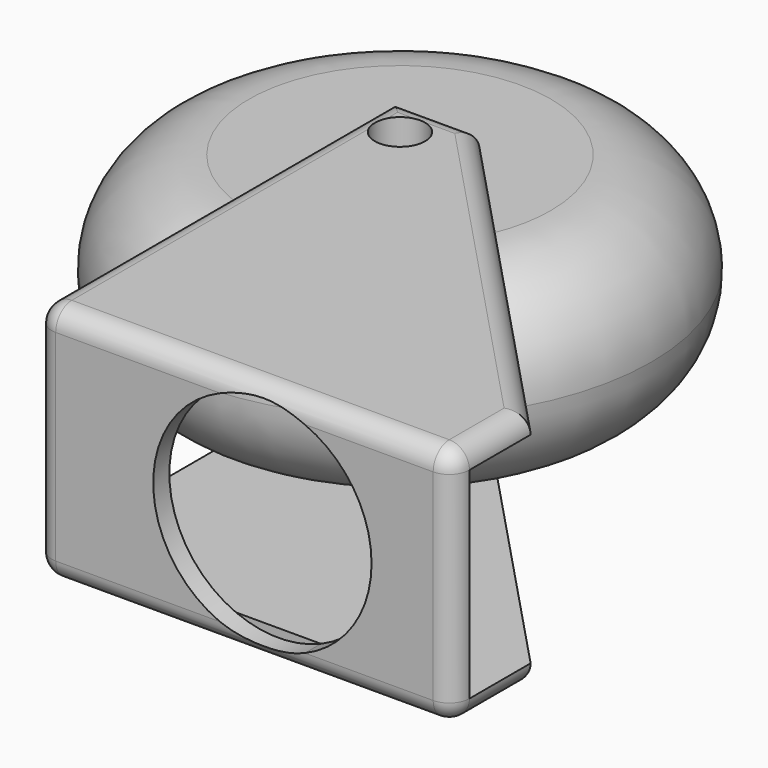
from build123d import *

# Parameters (mm, degrees)
F0_R          = 25
F1_DEPTH      = 20
F2_R          = 9.99999
F3_R          = 2.5
F4_DEPTH      = 25.4
F5_R          = 2.5
F6_DEPTH      = 2
F7_W          = 41.5132804774
F7_H          = 2
F8_DEPTH      = 20
F9_R          = 2.5
F9_W          = 41.5132804774
F9_H          = 2
F10_DEPTH     = 2
F11_T1_DEPTH  = 20
F11_T3_DEPTH  = 47.4638193212
F11_T5_DEPTH  = 37.5132804774
F11_T7_DEPTH  = 12.6040666103
F11_T9_DEPTH  = 57.9730332998
F11_T11_DEPTH = 18.5555869155
F11_T13_DEPTH = 57.9730332998
F11_S17_W     = 2
F11_S17_H     = 2
F11_T18_DEPTH = 2
F11_S23_W     = 2
F11_S23_H     = 2
F11_T24_DEPTH = 2
F11_S29_W     = 2
F11_S29_H     = 2
F11_T30_DEPTH = 2
F11_S35_W     = 2
F11_S35_H     = 2
F11_T36_DEPTH = 2
F13_DEPTH     = 2


# Not quite as in the source:
# - a fillet or chamfer that OpenCascade refuses, or shapes differently, is made with other operations: its cross-section is extruded or revolved along the edge and cut away or added
# - a fillet or chamfer is up to 0.001 mm smaller than in the source, because OpenCascade refuses the exact size


with BuildPart() as f1:
    # F0 (on Top) → F1 (new body)
    with BuildSketch(Plane.XY):
        Circle(F0_R)
    extrude(amount=F1_DEPTH)

    # F2 (radius 10 in the source; OpenCascade refuses exactly that, so slightly less here)
    f2_edges = [f1.edges().sort_by_distance(p)[0] for p in [
        (-25, 0, 20),
        (-25, 0, 0),
    ]]
    fillet(f2_edges, radius=F2_R)

    # F3 (on face) → F4 (cut)
    with BuildSketch(Plane.XY.offset(20)):
        Circle(F3_R)
    extrude(amount=-F4_DEPTH, mode=Mode.SUBTRACT)

    # F5 (on face) → F6 (join)
    with BuildSketch(Plane(origin=(0, 0, 0), x_dir=(1, 0, 0), z_dir=(0, 0, -1))):
        with BuildLine():
            Line((37.3017899692, 30.3959333897), (37.3017899692, 40))
            Line((37.3017899692, 40), (-4.2114905082, 40))
            Line((-4.2114905082, 40), (-4.2114905082, 14.3966540453))
            ThreePointArc((-4.2114905082, 14.3966540453), (6.5284436355, 13.5048037268), (13.8984988304, 5.641988148))
            Line((13.8984988304, 5.641988148), (37.3017899692, 30.3959333897))
        make_face()
        with BuildLine():
            Line((4.3440964073, -4.4638193212), (13.8984988304, 5.641988148))
            ThreePointArc((13.8984988304, 5.641988148), (6.5284436355, 13.5048037268), (-4.2114905082, 14.3966540453))
            Line((-4.2114905082, 14.3966540453), (-4.2114905082, -4.4638193212))
            Line((-4.2114905082, -4.4638193212), (4.3440964073, -4.4638193212))
        make_face()
        Circle(F5_R, mode=Mode.SUBTRACT)
    extrude(amount=F6_DEPTH)

    # F7 (on face) → F8 (join)
    with BuildSketch(Plane.XY):
        with Locations((16.5451497305, -39)):
            Rectangle(F7_W, F7_H)
    extrude(amount=F8_DEPTH)

    # F9 (on face) → F10 (join)
    with BuildSketch(Plane.XY.offset(20)):
        Polygon((37.3017899692, -38), (37.3017899692, -30.3959333897), (4.3440964073, 4.4638193212), (-4.2114905082, 4.4638193212), (-4.2114905082, -38), align=None)
        Circle(F9_R, mode=Mode.SUBTRACT)
        with Locations((16.5451497305, -39)):
            Rectangle(F9_W, F9_H)
    extrude(amount=F10_DEPTH)

    # F11: fillet of radius 2 on 12 edges, made by hand

    # F11_s2 → F11_t1 (cut)
    with BuildSketch(Plane.XY):
        with BuildLine():
            ThreePointArc((-2.2114905082, -40), (-3.6257040705, -39.4142135624), (-4.2114905082, -38))
            Line((-4.2114905082, -38), (-4.2114905082, -40))
            Line((-4.2114905082, -40), (-2.2114905082, -40))
        make_face()
        with BuildLine():
            ThreePointArc((35.3017899692, -40), (36.7160035316, -39.4142135624), (37.3017899692, -38))
            Line((37.3017899692, -38), (37.3017899692, -40))
            Line((37.3017899692, -40), (35.3017899692, -40))
        make_face()
    extrude(amount=F11_T1_DEPTH, mode=Mode.SUBTRACT)

    # F11_s4 → F11_t3 (cut)
    with BuildSketch(Plane.XZ.offset(-9.4638193212)):
        with BuildLine():
            ThreePointArc((-2.2114905082, 22), (-3.6257040705, 21.4142135624), (-4.2114905082, 20))
            Line((-4.2114905082, 20), (-4.2114905082, 22))
            Line((-4.2114905082, 22), (-2.2114905082, 22))
        make_face()
        with BuildLine():
            ThreePointArc((-2.2114905082, -2), (-3.6257040705, -1.4142135624), (-4.2114905082, 0))
            Line((-4.2114905082, 0), (-4.2114905082, -2))
            Line((-4.2114905082, -2), (-2.2114905082, -2))
        make_face()
    extrude(amount=F11_T3_DEPTH, mode=Mode.SUBTRACT)

    # F11_s6 → F11_t5 (cut)
    with BuildSketch(Plane.YZ.offset(-2.2114905082)):
        with BuildLine():
            ThreePointArc((-38, 22), (-39.4142135624, 21.4142135624), (-40, 20))
            Line((-40, 20), (-40, 22))
            Line((-40, 22), (-38, 22))
        make_face()
        with BuildLine():
            ThreePointArc((-38, -2), (-39.4142135624, -1.4142135624), (-40, 0))
            Line((-40, 0), (-40, -2))
            Line((-40, -2), (-38, -2))
        make_face()
    extrude(amount=F11_T5_DEPTH, mode=Mode.SUBTRACT)

    # F11_s8 → F11_t7 (cut)
    with BuildSketch(Plane.XZ.offset(25.3959333897)):
        with BuildLine():
            ThreePointArc((35.3017899692, 22), (36.7160035316, 21.4142135624), (37.3017899692, 20))
            Line((37.3017899692, 20), (37.3017899692, 22))
            Line((37.3017899692, 22), (35.3017899692, 22))
        make_face()
        with BuildLine():
            ThreePointArc((35.3017899692, -2), (36.7160035316, -1.4142135624), (37.3017899692, 0))
            Line((37.3017899692, 0), (37.3017899692, -2))
            Line((37.3017899692, -2), (35.3017899692, -2))
        make_face()
    extrude(amount=F11_T7_DEPTH, mode=Mode.SUBTRACT)

    # F11_s10 → F11_t9 (cut)
    with BuildSketch(Plane(origin=(36.2146215396, -38.3046449843, 0), x_dir=(0, 0, 1), z_dir=(-0.6870045793, 0.7266530864, 0))):
        with BuildLine():
            ThreePointArc((20, 6.223315377), (21.4142135624, 5.6375289394), (22, 4.223315377))
            Line((22, 4.223315377), (22, 6.223315377))
            Line((22, 6.223315377), (20, 6.223315377))
        make_face()
    extrude(amount=F11_T9_DEPTH, mode=Mode.SUBTRACT)

    # F11_s12 → F11_t11 (cut)
    with BuildSketch(Plane.YZ.offset(-9.2114905082)):
        with BuildLine():
            ThreePointArc((2.4638193212, 22), (3.8780328836, 21.4142135624), (4.4638193212, 20))
            Line((4.4638193212, 20), (4.4638193212, 22))
            Line((4.4638193212, 22), (2.4638193212, 22))
        make_face()
        with BuildLine():
            ThreePointArc((2.4638193212, -2), (3.8780328836, -1.4142135624), (4.4638193212, 0))
            Line((4.4638193212, 0), (4.4638193212, -2))
            Line((4.4638193212, -2), (2.4638193212, -2))
        make_face()
    extrude(amount=F11_T11_DEPTH, mode=Mode.SUBTRACT)

    # F11_s14 → F11_t13 (cut)
    with BuildSketch(Plane(origin=(-3.6131178157, 3.8216385905, 0), x_dir=(0, 0, 1), z_dir=(0.6870045793, -0.7266530864, 0))):
        with BuildLine():
            ThreePointArc((-2, -4.223315377), (-1.4142135624, -5.6375289394), (0, -6.223315377))
            Line((0, -6.223315377), (-2, -6.223315377))
            Line((-2, -6.223315377), (-2, -4.223315377))
        make_face()
    extrude(amount=F11_T13_DEPTH, mode=Mode.SUBTRACT)


with BuildPart() as f11_tool16:
    # F11_s17 → F11_t18 (new body)
    with BuildSketch(Plane.XZ.offset(38)):
        with Locations((-3.2114905082, -1)):
            Rectangle(F11_S17_W, F11_S17_H)
    extrude(amount=F11_T18_DEPTH)

    # F11_s19 → F11_t20 (revolve, cut)
    with BuildSketch(Plane(origin=(-2.2114905082, -38, 0), x_dir=(0.7071067812, 0, 0.7071067812), z_dir=(0.7071067812, 0, -0.7071067812))):
        with BuildLine():
            ThreePointArc((0, -2), (2, 0), (0, 2))
            Line((0, 2), (0, -2))
        make_face()
    revolve(axis=Axis((-2.2114905082, -38, 0), (0, -1, 0)), mode=Mode.SUBTRACT)


with BuildPart() as f1_1:
    add(f1.part)

    # F11_t15: cut F11_tool16
    add(f11_tool16.part, mode=Mode.SUBTRACT)


with BuildPart() as f11_tool22:
    # F11_s23 → F11_t24 (new body)
    with BuildSketch(Plane.XZ.offset(38)):
        with Locations((-3.2114905082, 21)):
            Rectangle(F11_S23_W, F11_S23_H)
    extrude(amount=F11_T24_DEPTH)

    # F11_s25 → F11_t26 (revolve, cut)
    with BuildSketch(Plane(origin=(-2.2114905082, -38, 20), x_dir=(0.7071067812, 0, -0.7071067812), z_dir=(-0.7071067812, 0, -0.7071067812))):
        with BuildLine():
            ThreePointArc((0, -2), (2, 0), (0, 2))
            Line((0, 2), (0, -2))
        make_face()
    revolve(axis=Axis((-2.2114905082, -38, 20), (0, -1, 0)), mode=Mode.SUBTRACT)


with BuildPart() as f1_2:
    add(f1_1.part)

    # F11_t21: cut F11_tool22
    add(f11_tool22.part, mode=Mode.SUBTRACT)


with BuildPart() as f11_tool28:
    # F11_s29 → F11_t30 (new body)
    with BuildSketch(Plane.XZ.offset(38)):
        with Locations((36.3017899692, 21)):
            Rectangle(F11_S29_W, F11_S29_H)
    extrude(amount=F11_T30_DEPTH)

    # F11_s31 → F11_t32 (revolve, cut)
    with BuildSketch(Plane(origin=(35.3017899692, -38, 20), x_dir=(-0.7071067812, 0, -0.7071067812), z_dir=(-0.7071067812, 0, 0.7071067812))):
        with BuildLine():
            ThreePointArc((0, -2), (2, 0), (0, 2))
            Line((0, 2), (0, -2))
        make_face()
    revolve(axis=Axis((35.3017899692, -38, 20), (0, -1, 0)), mode=Mode.SUBTRACT)


with BuildPart() as f1_3:
    add(f1_2.part)

    # F11_t27: cut F11_tool28
    add(f11_tool28.part, mode=Mode.SUBTRACT)


with BuildPart() as f11_tool34:
    # F11_s35 → F11_t36 (new body)
    with BuildSketch(Plane.XZ.offset(38)):
        with Locations((36.3017899692, -1)):
            Rectangle(F11_S35_W, F11_S35_H)
    extrude(amount=F11_T36_DEPTH)

    # F11_s37 → F11_t38 (revolve, cut)
    with BuildSketch(Plane(origin=(35.3017899692, -38, 0), x_dir=(-0.7071067812, 0, 0.7071067812), z_dir=(0.7071067812, 0, 0.7071067812))):
        with BuildLine():
            ThreePointArc((0, -2), (2, 0), (0, 2))
            Line((0, 2), (0, -2))
        make_face()
    revolve(axis=Axis((35.3017899692, -38, 0), (0, -1, 0)), mode=Mode.SUBTRACT)


with BuildPart() as f1_4:
    add(f1_3.part)

    # F11_t33: cut F11_tool34
    add(f11_tool34.part, mode=Mode.SUBTRACT)

    # F12 (on face) → F13 (cut)
    with BuildSketch(Plane.XZ.offset(40)):
        with BuildLine():
            Line((14.1298108305, 20), (22.5242070351, 20))
            ThreePointArc((22.5242070351, 20), (18.3270089328, 20.8447), (14.1298108305, 20))
        make_face()
        with BuildLine():
            ThreePointArc((22.5493864515, 0), (27.3695554789, 3.9984635169), (29.1770089328, 9.9947))
            ThreePointArc((29.1770089328, 9.9947), (27.3619992319, 16.0023160243), (22.5242070351, 20))
            Line((22.5242070351, 20), (14.1298108305, 20))
            ThreePointArc((14.1298108305, 20), (7.4770175315, 10.0083598225), (14.1046314142, 0))
            Line((14.1046314142, 0), (22.5493864515, 0))
        make_face()
        with BuildLine():
            ThreePointArc((14.1046314142, 0), (18.3270089328, -0.8553), (22.5493864515, 0))
            Line((22.5493864515, 0), (14.1046314142, 0))
        make_face()
    extrude(amount=-F13_DEPTH, mode=Mode.SUBTRACT)


solid = f1_4.part
